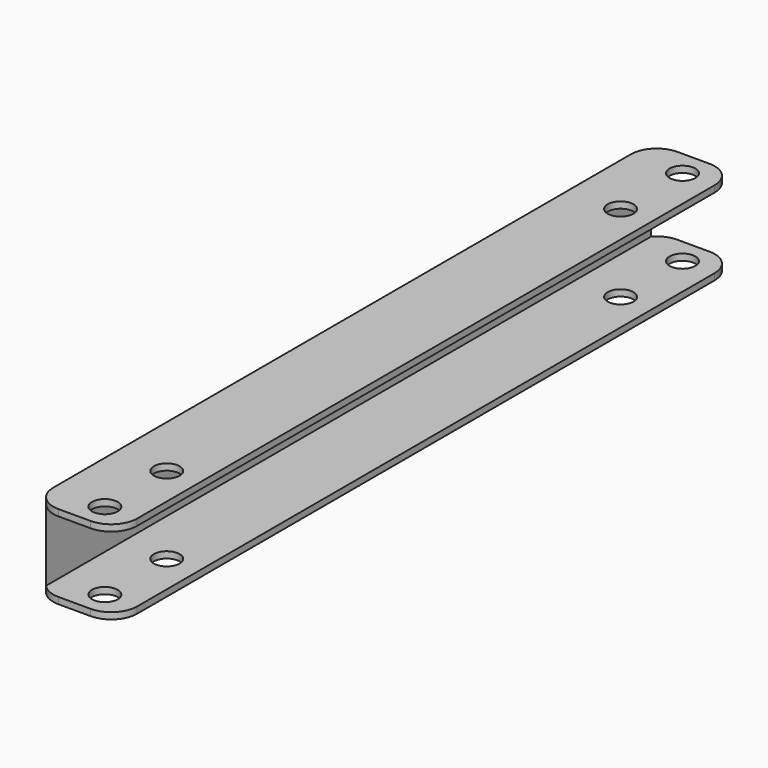
from build123d import *

# Parameters (mm, degrees)
F2_DEPTH    = 300
F1_R        = 5
F3_DEPTH    = 46
F4_T1_DEPTH = 52.5
F4_T3_DEPTH = 52.5
F4_T5_DEPTH = 82.5


# Not quite as in the source:
# - a fillet or chamfer that OpenCascade refuses, or shapes differently, is made with other operations: its cross-section is extruded or revolved along the edge and cut away or added


with BuildPart() as f2:
    # F0 (on Front) → F2 (new body)
    with BuildSketch(Plane.XZ):
        Polygon((-74.9858543277, 32.5), (-74.9858543277, 0), (-42.4858543277, 0), (-42.4858543277, 2.5), (-72.4858543277, 2.5), (-72.4858543277, 30), (-42.4858543277, 30), (-42.4858543277, 32.5), align=None)
    extrude(amount=F2_DEPTH)

    # F1 (on Top) → F3 (cut)
    with BuildSketch(Plane.XY):
        with BuildLine():
            ThreePointArc((-59.9858543277, -290), (-54.9858543277, -295), (-49.9858543277, -290))
            ThreePointArc((-49.9858543277, -290), (-54.9858543277, -285), (-59.9858543277, -290))
        make_face()
        with Locations((-54.9858543277, -260)):
            Circle(F1_R)
        with Locations((-54.9858543277, -40)):
            Circle(F1_R)
        with Locations((-54.9858543277, -10)):
            Circle(F1_R)
    extrude(amount=F3_DEPTH, mode=Mode.SUBTRACT)

    # F4: fillet of radius 10 on 6 edges, made by hand

    # F4_s2 → F4_t1 (cut)
    with BuildSketch(Plane.XY.offset(-25)):
        with BuildLine():
            ThreePointArc((-52.4858543277, 0), (-45.4147865158, -2.9289321881), (-42.4858543277, -10))
            Line((-42.4858543277, -10), (-42.4858543277, 0))
            Line((-42.4858543277, 0), (-52.4858543277, 0))
        make_face()
        with BuildLine():
            ThreePointArc((-52.4858543277, -300), (-45.4147865158, -297.0710678119), (-42.4858543277, -290))
            Line((-42.4858543277, -290), (-42.4858543277, -300))
            Line((-42.4858543277, -300), (-52.4858543277, -300))
        make_face()
    extrude(amount=F4_T1_DEPTH, mode=Mode.SUBTRACT)

    # F4_s4 → F4_t3 (cut)
    with BuildSketch(Plane.XY.offset(5)):
        with BuildLine():
            ThreePointArc((-42.4858543277, -10), (-45.4147865158, -2.9289321881), (-52.4858543277, 0))
            Line((-52.4858543277, 0), (-42.4858543277, 0))
            Line((-42.4858543277, 0), (-42.4858543277, -10))
        make_face()
        with BuildLine():
            ThreePointArc((-42.4858543277, -290), (-45.4147865158, -297.0710678119), (-52.4858543277, -300))
            Line((-52.4858543277, -300), (-42.4858543277, -300))
            Line((-42.4858543277, -300), (-42.4858543277, -290))
        make_face()
    extrude(amount=F4_T3_DEPTH, mode=Mode.SUBTRACT)

    # F4_s6 → F4_t5 (cut)
    with BuildSketch(Plane.XY.offset(-25)):
        with BuildLine():
            ThreePointArc((-64.9858543277, 0), (-72.0569221395, -2.9289321881), (-74.9858543277, -10))
            Line((-74.9858543277, -10), (-74.9858543277, 0))
            Line((-74.9858543277, 0), (-64.9858543277, 0))
        make_face()
        with BuildLine():
            ThreePointArc((-64.9858543277, -300), (-72.0569221395, -297.0710678119), (-74.9858543277, -290))
            Line((-74.9858543277, -290), (-74.9858543277, -300))
            Line((-74.9858543277, -300), (-64.9858543277, -300))
        make_face()
    extrude(amount=F4_T5_DEPTH, mode=Mode.SUBTRACT)


solid = f2.part
